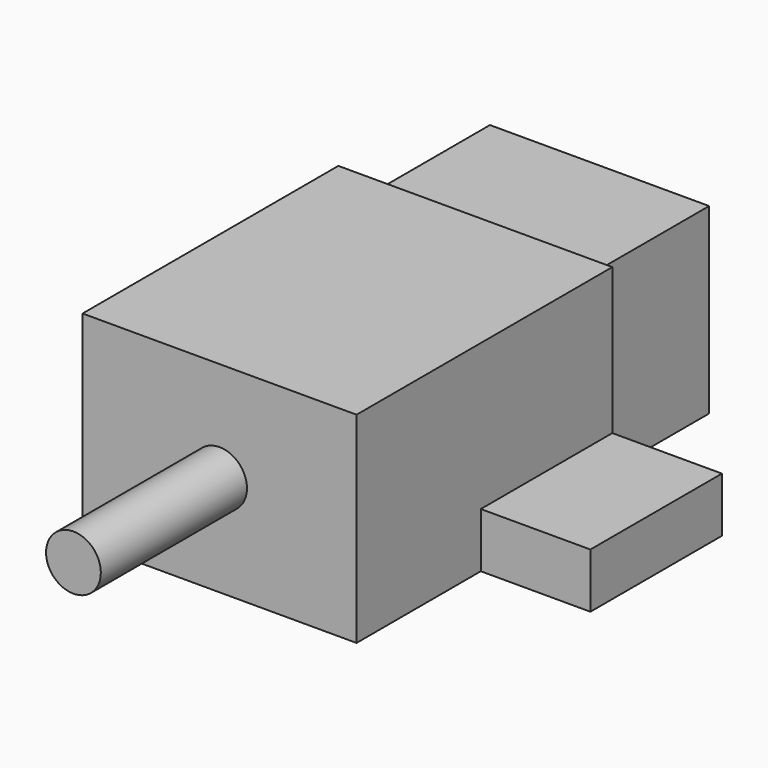
from build123d import *

# Parameters (mm, degrees)
F0_W     = 12
F0_H     = 26
F1_DEPTH = 10
F2_W     = 15
F2_H     = 17.5
F3_DEPTH = 11
F4_W     = 9
F4_H     = 3
F5_DEPTH = 6
F6_W     = 9
F6_H     = 3
F7_DEPTH = 6
F8_R     = 1.5
F9_DEPTH = 10


# Not quite as in the source:
# - a feature names something its author has since deleted; it is built from what else it names


with BuildPart() as f1:
    # F0 (on Top) → F1 (new body)
    with BuildSketch(Plane.XY):
        with Locations((0, 13)):
            Rectangle(F0_W, F0_H)
    extrude(amount=F1_DEPTH)

    # F2 (on Top) → F3 (join)
    with BuildSketch(Plane.XY):
        with Locations((0, 8.75)):
            Rectangle(F2_W, F2_H)
    extrude(amount=F3_DEPTH)

    # F4 (on face) → F5 (join)
    with BuildSketch(Plane.YZ.offset(7.5)):
        with Locations((13, 1.5)):
            Rectangle(F4_W, F4_H)
    extrude(amount=F5_DEPTH)

    # F6 (on face) → F7 (join)
    with BuildSketch(Plane(origin=(-7.5, 0, 0), x_dir=(0, -1, 0), z_dir=(-1, 0, 0))):
        with Locations((-13, 1.5)):
            Rectangle(F6_W, F6_H)
    extrude(amount=F7_DEPTH)

    # F8 (on face) → F9 (join)
    with BuildSketch(Plane.XZ):
        with Locations((0, 5.5)):
            Circle(F8_R)
    extrude(amount=F9_DEPTH)


solid = f1.part
